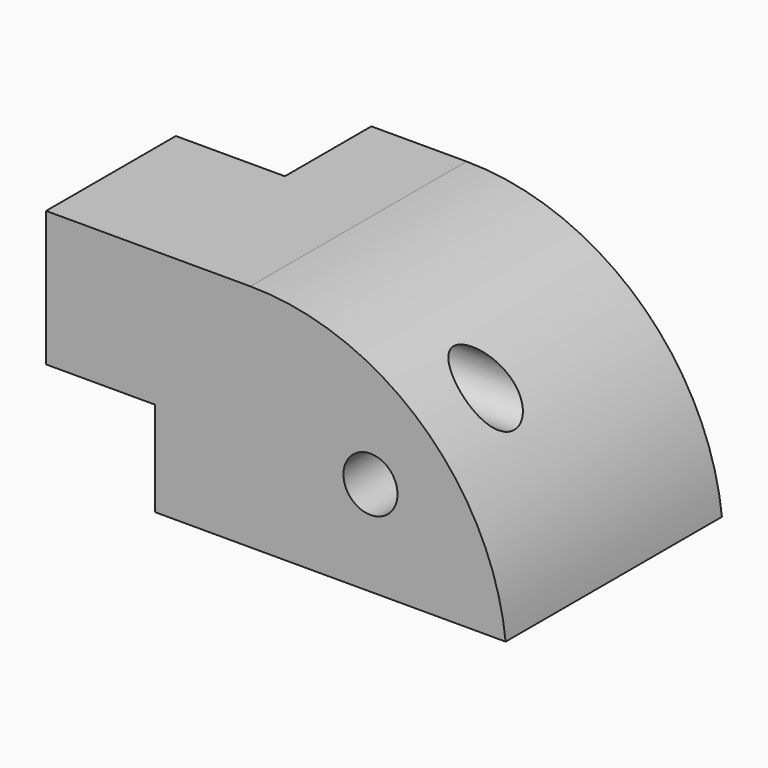
from build123d import *

# Parameters (mm, degrees)
F0_W        = 215.9
F0_H        = 127
F1_DEPTH    = 107.95
F4_W        = 50.8
F4_H        = 50.8
F5_DEPTH    = 107.95
F6_DEPTH    = 51.21156
F7_T1_DEPTH = 726.8985851792
F9_D        = 25.4
F10_D       = 25.4


# Not quite as in the source:
# - a fillet or chamfer that OpenCascade refuses, or shapes differently, is made with other operations: its cross-section is extruded or revolved along the edge and cut away or added


with BuildPart() as f1:
    # F0 (on Top) → F1 (new body)
    with BuildSketch(Plane.XY):
        with Locations((-26.1275832451, 6.2899636105)):
            Rectangle(F0_W, F0_H)
    extrude(amount=F1_DEPTH)

    # F4 (on face) → F5 (cut)
    with BuildSketch(Plane.XY.offset(107.95)):
        with Locations((-108.6775832451, 44.3899636105)):
            Rectangle(F4_W, F4_H)
    extrude(amount=-F5_DEPTH, mode=Mode.SUBTRACT)

    # F2 (on face) → F6 (cut)
    with BuildSketch(Plane(origin=(-134.0775832451, 0, 0), x_dir=(0, -1, 0), z_dir=(-1, 0, 0))):
        Polygon((-18.9899636105, 44.45), (-18.9899636105, 107.95), (-69.7899636105, 107.95), (-69.7899636105, 0), (57.2100363895, 0), (57.2100363895, 44.45), align=None)
    extrude(amount=-F6_DEPTH, mode=Mode.SUBTRACT)

    # F7: fillet of radius 120.65 on 1 edges, made by hand

    # F7_s2 → F7_t1 (cut)
    with BuildSketch(Plane.XZ.offset(-369.7392562001)):
        with BuildLine():
            ThreePointArc((81.8224167549, 0), (42.5401826414, 76.9902377631), (-38.1573002809, 107.95))
            Line((-38.1573002809, 107.95), (81.8224167549, 107.95))
            Line((81.8224167549, 107.95), (81.8224167549, 0))
        make_face()
    extrude(amount=F7_T1_DEPTH, mode=Mode.SUBTRACT)

    # F9 (through all)
    with Locations(Plane.XZ.offset(57.2100363895)):
        with Locations((18.3224167549, 44.45)):
            Hole(F9_D / 2)

    # F10 (through all)
    with Locations(Plane(origin=(-134.0775832451, 0, 0), x_dir=(0, -1, 0), z_dir=(-1, 0, 0))):
        with Locations((19.1100363895, 76.2)):
            Hole(F10_D / 2)


solid = f1.part
